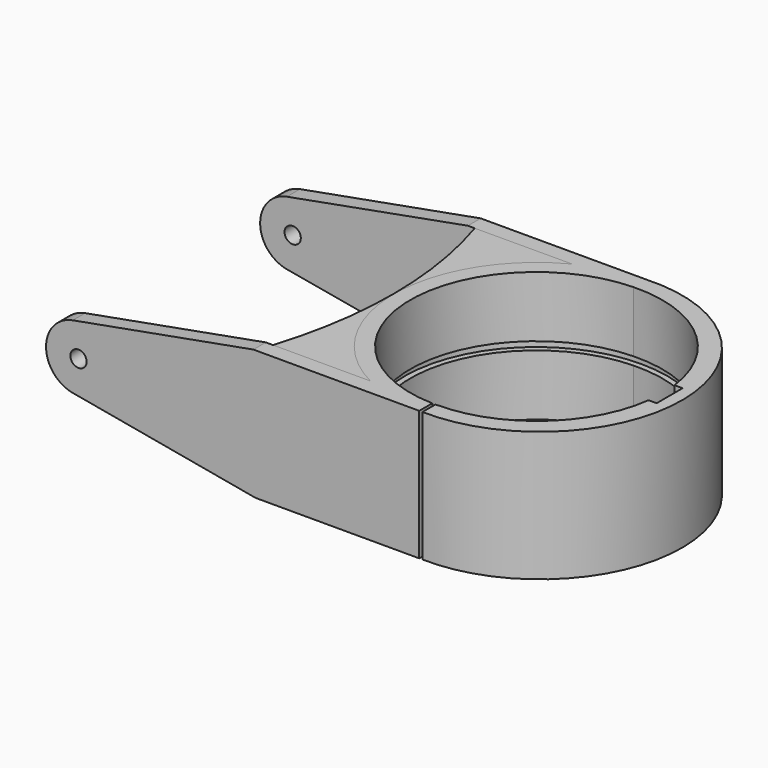
from build123d import *

# Parameters (mm, degrees)
F1_DEPTH  = 25.4
F3_DEPTH  = 25.4
F4_DEPTH  = 25.4
F7_DEPTH  = 120.65
F8_R      = 3.175
F9_DEPTH  = 114.3
F10_R     = 51.4598077904
F11_DEPTH = 1.5875
F12_T     = 2.54
F13_R     = 7.2100131565
F14_DEPTH = 20.32
F15_R     = 8.3028862555
F16_DEPTH = 17.78


# Not quite as in the source:
# - a shell that OpenCascade refuses in one call is made with other operations: the cavity is built on its own and cut out
# - the program builds the solid bodies; features that only make, move or delete a surface that nothing else refers to are left out


with BuildPart() as f1:
    # F0 (on Top) → F1 (new body, symmetric)
    with BuildSketch(Plane.XY):
        with BuildLine():
            ThreePointArc((-1.2680592233, -49.1961602369), (-49.2125, 0), (-1.2680592233, 49.1961602369))
            Line((-1.2680592233, 49.1961602369), (-1.2680592233, 55.5480281563))
            Line((-1.2680592233, 55.5480281563), (-147.3180592233, 55.5480281563))
            Line((-147.3180592233, 55.5480281563), (-147.3180592233, 49.091055685))
            Line((-147.3180592233, 49.091055685), (-63.4814364191, 49.3103835326))
            Line((-63.4814364191, 49.3103835326), (-25.4134971885, 49.4099743665))
            ThreePointArc((-25.4134971885, 49.4099743665), (-55.5624058885, -0.1022650226), (-25.2314432137, -49.5031885802))
            Line((-25.2314432137, -49.5031885802), (-63.3314432137, -49.5031885802))
            Line((-63.3314432137, -49.5031885802), (-69.6814432137, -49.5031885802))
            Line((-69.6814432137, -49.5031885802), (-147.3180592233, -49.5031885802))
            Line((-147.3180592233, -49.5031885802), (-147.3180592233, -55.5800534785))
            Line((-147.3180592233, -55.5800534785), (-1.2680592233, -55.5800534785))
            Line((-1.2680592233, -55.5800534785), (-1.2680592233, -49.1961602369))
        make_face()
    extrude(amount=F1_DEPTH, both=True)

    # F0 (on Top) → F4 (join, symmetric)
    with BuildSketch(Plane.XY):
        with BuildLine():
            ThreePointArc((49.0389416617, -6.35), (32.6236991353, -37.0532891725), (0, -49.2125))
            Line((0, -49.2125), (0, -55.5625))
            ThreePointArc((0, -55.5625), (57.0543020001, 0.6511375212), (-1.2680592233, 55.5480281563))
            Line((-1.2680592233, 55.5480281563), (-1.2680592233, 49.1961602369))
            ThreePointArc((-1.2680592233, 49.1961602369), (32.1458766832, 37.4716025001), (49.0397283671, 6.35))
            Line((49.0397283671, 6.35), (52.2147283671, 6.35))
            Line((52.2147283671, 6.35), (52.2147283671, -6.35))
            Line((52.2147283671, -6.35), (49.0389416617, -6.35))
        make_face()
    extrude(amount=F4_DEPTH, both=True)

    # F6 (on face) → F7 (cut)
    with BuildSketch(Plane.XZ.offset(55.5800534785)):
        with BuildLine():
            ThreePointArc((-137.0693669386, -12.441398865), (-147.2188088745, 0.1366940896), (-136.8009702954, 12.493402119))
            Line((-136.8009702954, 12.493402119), (-66.122660171, 25.4))
            Line((-66.122660171, 25.4), (-147.3180592233, 25.4))
            Line((-147.3180592233, 25.4), (-147.3180592233, -25.4))
            Line((-147.3180592233, -25.4), (-65.2581656686, -25.4))
            Line((-65.2581656686, -25.4), (-137.0693669386, -12.441398865))
        make_face()
    extrude(amount=-F7_DEPTH, mode=Mode.SUBTRACT)

    # F8 (on face) → F9 (cut)
    with BuildSketch(Plane(origin=(0, 55.5480281563, 0), x_dir=(-1, 0, 0), z_dir=(0, 1, 0))):
        with Locations((134.5195445365, 0)):
            Circle(F8_R)
    extrude(amount=-F9_DEPTH, mode=Mode.SUBTRACT)

    # F10 (on Top) → F11 (cut, symmetric)
    with BuildSketch(Plane.XY):
        Circle(F10_R)
    extrude(amount=F11_DEPTH, both=True, mode=Mode.SUBTRACT)

    # F13 (on face) → F14 (cut)
    with BuildSketch(Plane(origin=(0, 55.5480281563, 0), x_dir=(-1, 0, 0), z_dir=(0, 1, 0))):
        with Locations((48.4190694988, 0)):
            Circle(F13_R)
    extrude(amount=-F14_DEPTH, mode=Mode.SUBTRACT)


with BuildPart() as f3:
    # F0 (on Top) → F3 (new body, symmetric)
    with BuildSketch(Plane.XY):
        with BuildLine():
            Line((-25.4134971885, 49.4099743665), (-63.4814364191, 49.3103835326))
            ThreePointArc((-63.4814364191, 49.3103835326), (-55.6963964132, -0.0846991302), (-63.3314432137, -49.5031885802))
            Line((-63.3314432137, -49.5031885802), (-25.2314432137, -49.5031885802))
            ThreePointArc((-25.2314432137, -49.5031885802), (-55.5624058885, -0.1022650226), (-25.4134971885, 49.4099743665))
        make_face()
    extrude(amount=F3_DEPTH, both=True)

    # F12: shell of thickness 2.54, made by hand


with BuildPart() as f12_core1:
    # F12_t2: copy of F3
    add(f3.part)

    # the walls: a layer under each face that stays
    f12_faces = [f12_core1.faces().sort_by_distance(p)[0] for p in [
        (-44.2814432137, -49.5031885802, 0),
        (-44.4474668038, 49.3601789496, 0),
        (-57.1064375515, -33.0176614224, 25.4),
        (-55.5624058885, -0.1022650226, 0),
        (-57.1064375515, -33.0176614224, -25.4),
    ]]
    thicken(f12_faces, amount=-F12_T, mode=Mode.SUBTRACT)


with BuildPart() as f3_1:
    add(f3.part)

    # what is left inside the walls is the cavity
    f12_cavity = [f12_core1.part.solids().sort_by_distance(p)[0] for p in [
        (-48.126372, -32.599157, -7.62),
        (-48.23108, 32.444039, -7.62),
    ]]
    add(f12_cavity, mode=Mode.SUBTRACT)

    # F15 (on face) → F16 (cut)
    with BuildSketch(Plane(origin=(-0.122791209, 46.9361295528, 0), x_dir=(0.9999965779, 0.0026161251, 0), z_dir=(0.0026161251, -0.9999965779, 0))):
        with Locations((-48.4509207308, 0)):
            Circle(F15_R)
    extrude(amount=-F16_DEPTH, mode=Mode.SUBTRACT)


solid = Compound([f1.part, f3_1.part])
